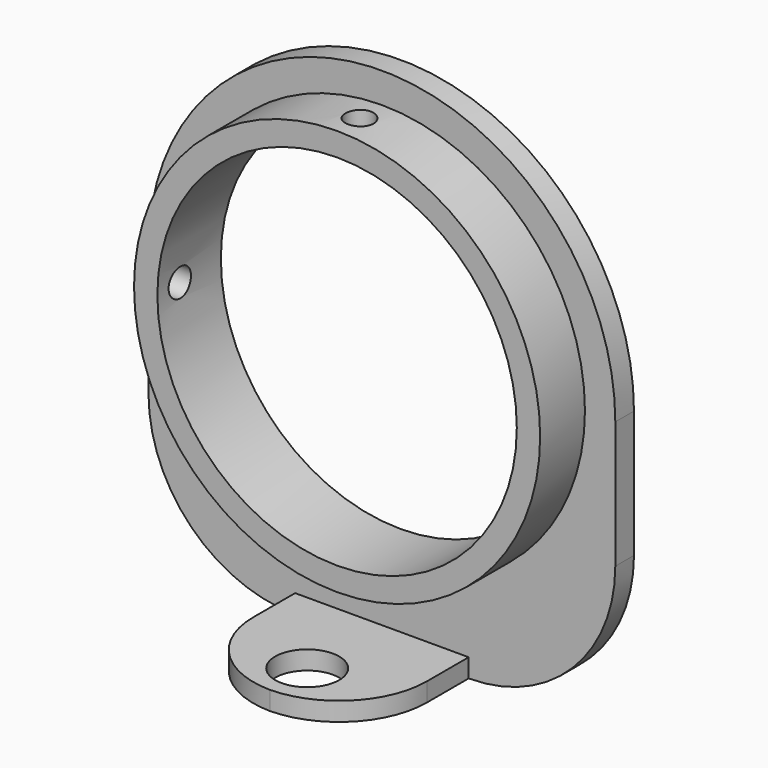
from build123d import *

# Parameters (mm, degrees)
F0_R            = 21.75
F0_R_2          = 19.25
F1_DEPTH        = 6
F3_DEPTH        = 2.5
F4_R            = 19.25
F5_DEPTH        = 25
F6_R            = 1.5
F7_DEPTH        = 25
F7_COPIES_COUNT = 2
F7_COPIES_ANGLE = 270
F8_W            = 18.5894630849
F8_H            = 2
F9_DEPTH        = 15
F10_R           = 15.6923881554
F11_T1_DEPTH    = 25.5385822331
F12_R           = 3.429
F13_DEPTH       = 25


# Not quite as in the source:
# - a fillet or chamfer that OpenCascade refuses, or shapes differently, is made with other operations: its cross-section is extruded or revolved along the edge and cut away or added
# - a pattern or mirror of a feature is missing from the dataset's text; its kind, count and spacing are read off the source's solid


with BuildPart() as f1:
    # F0 (on Front) → F1 (new body)
    with BuildSketch(Plane.XZ):
        Circle(F0_R)
        Circle(F0_R_2, mode=Mode.SUBTRACT)
    extrude(amount=F1_DEPTH)

    # F2 (on Front) → F3 (join)
    with BuildSketch(Plane.XZ):
        with BuildLine():
            ThreePointArc((-25, 0), (0, -25), (25, 0))
            ThreePointArc((25, 0), (0, 25), (-25, 0))
        make_face()
        with BuildLine():
            Line((25, -29.2988744574), (25, 0))
            ThreePointArc((25, 0), (0, -25), (-25, 0))
            Line((-25, 0), (-25, -29.2988744574))
            Line((-25, -29.2988744574), (25, -29.2988744574))
        make_face()
    extrude(amount=-F3_DEPTH)

    # F4 (on Front) → F5 (cut)
    with BuildSketch(Plane.XZ):
        Circle(F4_R)
    extrude(amount=-F5_DEPTH, mode=Mode.SUBTRACT)

    # F6 (on Top) → F7 (cut)
    with BuildSketch(Plane.XY):
        with Locations((0, -3)):
            Circle(F6_R)
    f7 = extrude(amount=F7_DEPTH, mode=Mode.SUBTRACT)

    # F7_copies: F7 ×2 about axis
    f7_copies_axis = Axis((0, 0, 0), (0, 1, 0))
    for i in range(1, F7_COPIES_COUNT):
        add(f7.rotate(f7_copies_axis, i * F7_COPIES_ANGLE / (F7_COPIES_COUNT - 1)), mode=Mode.SUBTRACT)

    # F8 (on face) → F9 (join)
    with BuildSketch(Plane.XZ):
        with Locations((0, -28.2988744574)):
            Rectangle(F8_W, F8_H)
    extrude(amount=F9_DEPTH)

    # F10
    f10_edges = [f1.edges().sort_by_distance(p)[0] for p in [
        (-25, 1.25, -29.298874),
        (25, 1.25, -29.298874),
    ]]
    fillet(f10_edges, radius=F10_R)

    # F11: fillet of radius 9.4154328933 on 2 edges, made by hand

    # F11_s2 → F11_t1 (cut)
    with BuildSketch(Plane.XY.offset(-52.8374566906)):
        with BuildLine():
            ThreePointArc((9.2947315425, -5.5845671067), (6.5370150958, -12.2422835534), (-0.1207013508, -15))
            Line((-0.1207013508, -15), (9.2947315425, -15))
            Line((9.2947315425, -15), (9.2947315425, -5.5845671067))
        make_face()
        with BuildLine():
            ThreePointArc((-9.2947315425, -5.5845671067), (-6.5370150958, -12.2422835534), (0.1207013508, -15))
            Line((0.1207013508, -15), (-9.2947315425, -15))
            Line((-9.2947315425, -15), (-9.2947315425, -5.5845671067))
        make_face()
    extrude(amount=F11_T1_DEPTH, mode=Mode.SUBTRACT)

    # F12 (on face) → F13 (cut)
    with BuildSketch(Plane.XY.offset(-27.2988744574)):
        with Locations((0, -9.9992263014)):
            Circle(F12_R)
    extrude(amount=-F13_DEPTH, mode=Mode.SUBTRACT)


solid = f1.part
